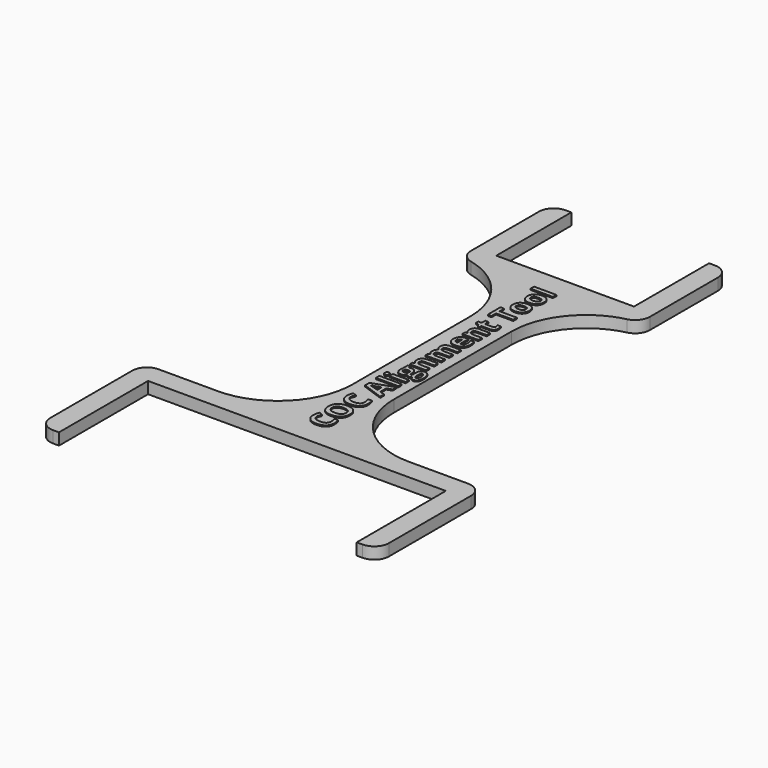
from build123d import *

# Parameters (mm, degrees)
F1_DEPTH     = 4
F2_R         = 5
F3_R         = 25.4878494875
F4_TEXT_SIZE = 10.0334961063
F5_DEPTH     = 0.4


# Not quite as in the source:
# - Text() gives the source's letters only with a copy of the font that has no kerning and outlines rounded to 1/6400 em; it was checked with that copy


with BuildPart() as f1:
    # F0 (on Top) → F1 (new body)
    with BuildSketch(Plane.XY):
        Polygon((-50.8, -95.2), (-50.8, -57.2), (50.8, -57.2), (50.8, -95.2), (57.8, -95.2), (57.8, -57.2), (57.8, -50.2), (22, -50.2), (7, -50.2), (7, -35.2), (7, 50.2), (30.5, 50.2), (30.5, 57.2), (30.5, 89.2), (23.5, 89.2), (23.5, 57.2), (-23.5, 57.2), (-23.5, 89.2), (-30.5, 89.2), (-30.5, 57.2), (-30.5, 50.2), (-7, 50.2), (-7, -35.2), (-7, -50.2), (-22, -50.2), (-57.8, -50.2), (-57.8, -57.2), (-57.8, -95.2), align=None)
        Polygon((-7, -35.2), (-22, -50.2), (-7, -50.2), align=None)
        Polygon((7, -50.2), (22, -50.2), (7, -35.2), align=None)
    extrude(amount=F1_DEPTH)

    # F2
    f2_edges = [f1.edges().sort_by_distance(p)[0] for p in [
        (-57.8, -50.2, 2),
        (57.8, -50.2, 2),
        (30.5, 50.2, 2),
        (-30.5, 50.2, 2),
        (-57.8, -95.2, 2),
        (57.8, -95.2, 2),
        (30.5, 89.2, 2),
        (-30.5, 89.2, 2),
    ]]
    fillet(f2_edges, radius=F2_R)

    # F3
    f3_edges = [f1.edges().sort_by_distance(p)[0] for p in [
        (-7, -35.2, 2),
        (-22, -50.2, 2),
        (22, -50.2, 2),
        (7, -35.2, 2),
        (-7, 50.2, 2),
        (7, 50.2, 2),
    ]]
    fillet(f3_edges, radius=F3_R)

    # F4 (on face) → F5 (join)
    with BuildSketch(Plane.XY.offset(4)):
        with Locations(Location((3.6120585983, -49.5944738397), (0, 0, 90))):
            Text('COC Alignment Tool', F4_TEXT_SIZE, font='Open Sans', font_style=FontStyle.BOLD, text_align=(TextAlign.LEFT, TextAlign.BOTTOM))
    extrude(amount=F5_DEPTH)


solid = f1.part
